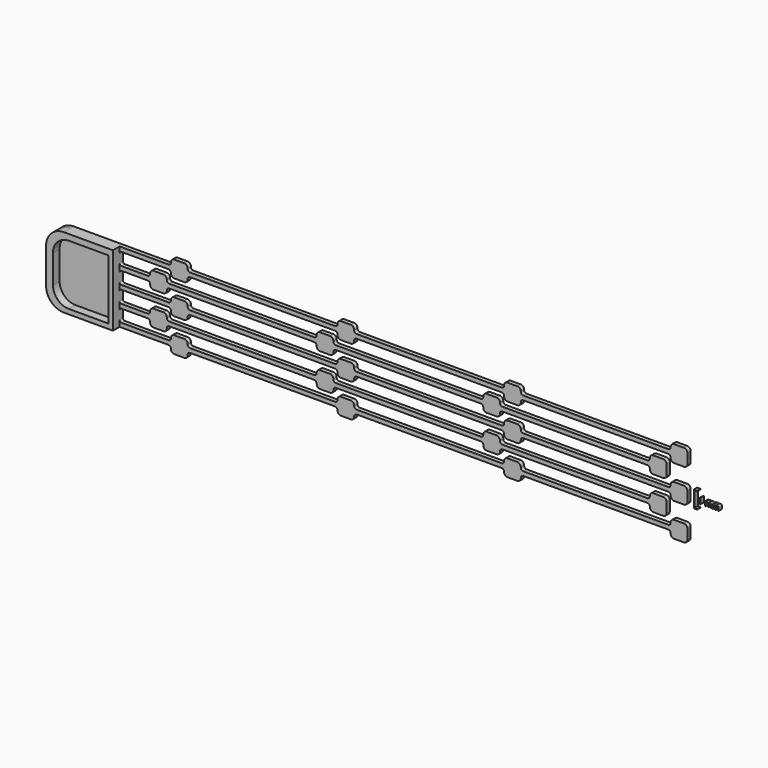
from build123d import *

# Parameters (mm, degrees)
F1_DEPTH     = 0.25
F2_W         = 0.0440478325
F2_H         = 0.0398103148
F2_W_2       = 0.1596286893
F2_H_2       = 0.9191203862
F2_H_3       = 0.0411942601
F2_TEXT_SIZE = 0.4795742118
F3_DEPTH     = 0.25
F5_DEPTH     = 0.5
F7_DEPTH     = 0.5


# Not quite as in the source:
# - ends of sketch curves that miss each other by under 0.0002 mm in the source are joined
# - Text() gives the source's letters only with a copy of the font that has no kerning and outlines rounded to 1/6400 em; it was checked with that copy


with BuildPart() as f1:
    # F0 (on Front) → F1 (new body)
    with BuildSketch(Plane.XZ):
        with BuildLine():
            ThreePointArc((50.7212476134, 27.8172210783), (50.6626689697, 27.9586424345), (50.5212476134, 28.0172210783))
            Line((50.5212476134, 28.0172210783), (49.9212476134, 28.0172210783))
            ThreePointArc((49.9212476134, 28.0172210783), (49.7798262572, 27.9586424345), (49.7212476134, 27.8172210783))
            Line((49.7212476134, 27.8172210783), (49.7212476134, 27.7922210783))
            ThreePointArc((49.7212476134, 27.7922210783), (49.6773136306, 27.6861550611), (49.5712476134, 27.6422210783))
            Line((49.5712476134, 27.6422210783), (49.1332476134, 27.6422210783))
            Line((49.1332476134, 27.6422210783), (47.8865653276, 27.6422210783))
            Line((47.8865653276, 27.6422210783), (46.7647824857, 27.6422210783))
            ThreePointArc((46.7647824857, 27.6422210783), (46.6741192638, 27.6797750144), (46.6365653276, 27.7704382363))
            Line((46.6365653276, 27.7704382363), (46.6365653276, 28.2640039202))
            ThreePointArc((46.6365653276, 28.2640039202), (46.6741192638, 28.3546671421), (46.7647824857, 28.3922210783))
            Line((46.7647824857, 28.3922210783), (47.8865653276, 28.3922210783))
            Line((47.8865653276, 28.3922210783), (48.3212476134, 28.3922210783))
            ThreePointArc((48.3212476134, 28.3922210783), (48.4273136306, 28.3482870955), (48.4712476134, 28.2422210783))
            Line((48.4712476134, 28.2422210783), (48.4712476134, 28.2172210783))
            ThreePointArc((48.4712476134, 28.2172210783), (48.5298262572, 28.075799722), (48.6712476134, 28.0172210783))
            Line((48.6712476134, 28.0172210783), (49.2712476134, 28.0172210783))
            ThreePointArc((49.2712476134, 28.0172210783), (49.4126689697, 28.075799722), (49.4712476134, 28.2172210783))
            Line((49.4712476134, 28.2172210783), (49.4712476134, 28.2422210783))
            ThreePointArc((49.4712476134, 28.2422210783), (49.5151815963, 28.3482870955), (49.6212476134, 28.3922210783))
            Line((49.6212476134, 28.3922210783), (51.1654019356, 28.3922210783))
            Line((51.1654019356, 28.3922210783), (57.8865653276, 28.3922210783))
            Line((57.8865653276, 28.3922210783), (58.3212476134, 28.3922210783))
            ThreePointArc((58.3212476134, 28.3922210783), (58.4273136306, 28.3482870955), (58.4712476134, 28.2422210783))
            Line((58.4712476134, 28.2422210783), (58.4712476134, 28.2172210783))
            ThreePointArc((58.4712476134, 28.2172210783), (58.5298262572, 28.075799722), (58.6712476134, 28.0172210783))
            Line((58.6712476134, 28.0172210783), (59.2712476134, 28.0172210783))
            ThreePointArc((59.2712476134, 28.0172210783), (59.4126689697, 28.075799722), (59.4712476134, 28.2172210783))
            Line((59.4712476134, 28.2172210783), (59.4712476134, 28.2422210783))
            ThreePointArc((59.4712476134, 28.2422210783), (59.5151815963, 28.3482870955), (59.6212476134, 28.3922210783))
            Line((59.6212476134, 28.3922210783), (61.1654019356, 28.3922210783))
            Line((61.1654019356, 28.3922210783), (67.8865653276, 28.3922210783))
            Line((67.8865653276, 28.3922210783), (68.3212476134, 28.3922210783))
            ThreePointArc((68.3212476134, 28.3922210783), (68.4273136306, 28.3482870955), (68.4712476134, 28.2422210783))
            Line((68.4712476134, 28.2422210783), (68.4712476134, 28.2172210783))
            ThreePointArc((68.4712476134, 28.2172210783), (68.5298262572, 28.075799722), (68.6712476134, 28.0172210783))
            Line((68.6712476134, 28.0172210783), (69.2712476134, 28.0172210783))
            ThreePointArc((69.2712476134, 28.0172210783), (69.4126689697, 28.075799722), (69.4712476134, 28.2172210783))
            Line((69.4712476134, 28.2172210783), (69.4712476134, 28.2422210783))
            ThreePointArc((69.4712476134, 28.2422210783), (69.5151815963, 28.3482870955), (69.6212476134, 28.3922210783))
            Line((69.6212476134, 28.3922210783), (71.1654019356, 28.3922210783))
            Line((71.1654019356, 28.3922210783), (77.8865653276, 28.3922210783))
            Line((77.8865653276, 28.3922210783), (78.3212476134, 28.3922210783))
            ThreePointArc((78.3212476134, 28.3922210783), (78.4273136306, 28.3482870955), (78.4712476134, 28.2422210783))
            Line((78.4712476134, 28.2422210783), (78.4712476134, 28.2172210783))
            ThreePointArc((78.4712476134, 28.2172210783), (78.5298262572, 28.075799722), (78.6712476134, 28.0172210783))
            Line((78.6712476134, 28.0172210783), (79.2712476134, 28.0172210783))
            ThreePointArc((79.2712476134, 28.0172210783), (79.4126689697, 28.075799722), (79.4712476134, 28.2172210783))
            Line((79.4712476134, 28.2172210783), (79.4712476134, 28.2422210783))
            Line((79.4712476134, 28.2422210783), (79.4712476134, 28.7922210783))
            Line((79.4712476134, 28.7922210783), (79.4712476134, 28.8172210783))
            ThreePointArc((79.4712476134, 28.8172210783), (79.4126689697, 28.9586424345), (79.2712476134, 29.0172210783))
            Line((79.2712476134, 29.0172210783), (78.6712476134, 29.0172210783))
            ThreePointArc((78.6712476134, 29.0172210783), (78.5298262572, 28.9586424345), (78.4712476134, 28.8172210783))
            Line((78.4712476134, 28.8172210783), (78.4712476134, 28.7922210783))
            ThreePointArc((78.4712476134, 28.7922210783), (78.4273136306, 28.6861550611), (78.3212476134, 28.6422210783))
            Line((78.3212476134, 28.6422210783), (77.8865653276, 28.6422210783))
            Line((77.8865653276, 28.6422210783), (71.1654019356, 28.6422210783))
            Line((71.1654019356, 28.6422210783), (69.6212476134, 28.6422210783))
            ThreePointArc((69.6212476134, 28.6422210783), (69.5151815963, 28.6861550611), (69.4712476134, 28.7922210783))
            Line((69.4712476134, 28.7922210783), (69.4712476134, 28.8172210783))
            ThreePointArc((69.4712476134, 28.8172210783), (69.4126689697, 28.9586424345), (69.2712476134, 29.0172210783))
            Line((69.2712476134, 29.0172210783), (68.6712476134, 29.0172210783))
            ThreePointArc((68.6712476134, 29.0172210783), (68.5298262572, 28.9586424345), (68.4712476134, 28.8172210783))
            Line((68.4712476134, 28.8172210783), (68.4712476134, 28.7922210783))
            ThreePointArc((68.4712476134, 28.7922210783), (68.4273136306, 28.6861550611), (68.3212476134, 28.6422210783))
            Line((68.3212476134, 28.6422210783), (67.8865653276, 28.6422210783))
            Line((67.8865653276, 28.6422210783), (61.1654019356, 28.6422210783))
            Line((61.1654019356, 28.6422210783), (59.6212476134, 28.6422210783))
            ThreePointArc((59.6212476134, 28.6422210783), (59.5151815963, 28.6861550611), (59.4712476134, 28.7922210783))
            Line((59.4712476134, 28.7922210783), (59.4712476134, 28.8172210783))
            ThreePointArc((59.4712476134, 28.8172210783), (59.4126689697, 28.9586424345), (59.2712476134, 29.0172210783))
            Line((59.2712476134, 29.0172210783), (58.6712476134, 29.0172210783))
            ThreePointArc((58.6712476134, 29.0172210783), (58.5298262572, 28.9586424345), (58.4712476134, 28.8172210783))
            Line((58.4712476134, 28.8172210783), (58.4712476134, 28.7922210783))
            ThreePointArc((58.4712476134, 28.7922210783), (58.4273136306, 28.6861550611), (58.3212476134, 28.6422210783))
            Line((58.3212476134, 28.6422210783), (57.8865653276, 28.6422210783))
            Line((57.8865653276, 28.6422210783), (51.1654019356, 28.6422210783))
            Line((51.1654019356, 28.6422210783), (49.6212476134, 28.6422210783))
            ThreePointArc((49.6212476134, 28.6422210783), (49.5151815963, 28.6861550611), (49.4712476134, 28.7922210783))
            Line((49.4712476134, 28.7922210783), (49.4712476134, 28.8172210783))
            ThreePointArc((49.4712476134, 28.8172210783), (49.4126689697, 28.9586424345), (49.2712476134, 29.0172210783))
            Line((49.2712476134, 29.0172210783), (48.6712476134, 29.0172210783))
            ThreePointArc((48.6712476134, 29.0172210783), (48.5298262572, 28.9586424345), (48.4712476134, 28.8172210783))
            Line((48.4712476134, 28.8172210783), (48.4712476134, 28.7922210783))
            ThreePointArc((48.4712476134, 28.7922210783), (48.4273136306, 28.6861550611), (48.3212476134, 28.6422210783))
            Line((48.3212476134, 28.6422210783), (47.8865653276, 28.6422210783))
            Line((47.8865653276, 28.6422210783), (46.7647824857, 28.6422210783))
            ThreePointArc((46.7647824857, 28.6422210783), (46.6741192638, 28.6797750144), (46.6365653276, 28.7704382363))
            Line((46.6365653276, 28.7704382363), (46.6365653276, 29.2640039202))
            ThreePointArc((46.6365653276, 29.2640039202), (46.6741192638, 29.3546671421), (46.7647824857, 29.3922210783))
            Line((46.7647824857, 29.3922210783), (47.8865653276, 29.3922210783))
            Line((47.8865653276, 29.3922210783), (49.1332476134, 29.3922210783))
            Line((49.1332476134, 29.3922210783), (49.5712476134, 29.3922210783))
            ThreePointArc((49.5712476134, 29.3922210783), (49.6773136306, 29.3482870955), (49.7212476134, 29.2422210783))
            Line((49.7212476134, 29.2422210783), (49.7212476134, 29.2172210783))
            ThreePointArc((49.7212476134, 29.2172210783), (49.7798262572, 29.075799722), (49.9212476134, 29.0172210783))
            Line((49.9212476134, 29.0172210783), (50.5212476134, 29.0172210783))
            ThreePointArc((50.5212476134, 29.0172210783), (50.6626689697, 29.075799722), (50.7212476134, 29.2172210783))
            Line((50.7212476134, 29.2172210783), (50.7212476134, 29.2422210783))
            ThreePointArc((50.7212476134, 29.2422210783), (50.7651815963, 29.3482870955), (50.8712476134, 29.3922210783))
            Line((50.8712476134, 29.3922210783), (51.1654019356, 29.3922210783))
            Line((51.1654019356, 29.3922210783), (57.8865653276, 29.3922210783))
            Line((57.8865653276, 29.3922210783), (59.1332476134, 29.3922210783))
            Line((59.1332476134, 29.3922210783), (59.5712476134, 29.3922210783))
            ThreePointArc((59.5712476134, 29.3922210783), (59.6773136306, 29.3482870955), (59.7212476134, 29.2422210783))
            Line((59.7212476134, 29.2422210783), (59.7212476134, 29.2172210783))
            ThreePointArc((59.7212476134, 29.2172210783), (59.7798262572, 29.075799722), (59.9212476134, 29.0172210783))
            Line((59.9212476134, 29.0172210783), (60.5212476134, 29.0172210783))
            ThreePointArc((60.5212476134, 29.0172210783), (60.6626689697, 29.075799722), (60.7212476134, 29.2172210783))
            Line((60.7212476134, 29.2172210783), (60.7212476134, 29.2422210783))
            ThreePointArc((60.7212476134, 29.2422210783), (60.7651815963, 29.3482870955), (60.8712476134, 29.3922210783))
            Line((60.8712476134, 29.3922210783), (61.1654019356, 29.3922210783))
            Line((61.1654019356, 29.3922210783), (67.8865653276, 29.3922210783))
            Line((67.8865653276, 29.3922210783), (69.1332476134, 29.3922210783))
            Line((69.1332476134, 29.3922210783), (69.5712476134, 29.3922210783))
            ThreePointArc((69.5712476134, 29.3922210783), (69.6773136306, 29.3482870955), (69.7212476134, 29.2422210783))
            Line((69.7212476134, 29.2422210783), (69.7212476134, 29.2172210783))
            ThreePointArc((69.7212476134, 29.2172210783), (69.7798262572, 29.075799722), (69.9212476134, 29.0172210783))
            Line((69.9212476134, 29.0172210783), (70.5212476134, 29.0172210783))
            ThreePointArc((70.5212476134, 29.0172210783), (70.6626689697, 29.075799722), (70.7212476134, 29.2172210783))
            Line((70.7212476134, 29.2172210783), (70.7212476134, 29.2422210783))
            ThreePointArc((70.7212476134, 29.2422210783), (70.7651815963, 29.3482870955), (70.8712476134, 29.3922210783))
            Line((70.8712476134, 29.3922210783), (71.1654019356, 29.3922210783))
            Line((71.1654019356, 29.3922210783), (77.8865653276, 29.3922210783))
            Line((77.8865653276, 29.3922210783), (79.1332476134, 29.3922210783))
            Line((79.1332476134, 29.3922210783), (79.5712476134, 29.3922210783))
            ThreePointArc((79.5712476134, 29.3922210783), (79.6773136306, 29.3482870955), (79.7212476134, 29.2422210783))
            Line((79.7212476134, 29.2422210783), (79.7212476134, 29.2172210783))
            ThreePointArc((79.7212476134, 29.2172210783), (79.7798262572, 29.075799722), (79.9212476134, 29.0172210783))
            Line((79.9212476134, 29.0172210783), (80.5212476134, 29.0172210783))
            ThreePointArc((80.5212476134, 29.0172210783), (80.6626689697, 29.075799722), (80.7212476134, 29.2172210783))
            Line((80.7212476134, 29.2172210783), (80.7212476134, 29.2422210783))
            Line((80.7212476134, 29.2422210783), (80.7212476134, 29.7922210783))
            Line((80.7212476134, 29.7922210783), (80.7212476134, 29.8172210783))
            ThreePointArc((80.7212476134, 29.8172210783), (80.6626689697, 29.9586424345), (80.5212476134, 30.0172210783))
            Line((80.5212476134, 30.0172210783), (79.9212476134, 30.0172210783))
            ThreePointArc((79.9212476134, 30.0172210783), (79.7798262572, 29.9586424345), (79.7212476134, 29.8172210783))
            Line((79.7212476134, 29.8172210783), (79.7212476134, 29.7922210783))
            ThreePointArc((79.7212476134, 29.7922210783), (79.6773136306, 29.6861550611), (79.5712476134, 29.6422210783))
            Line((79.5712476134, 29.6422210783), (79.1332476134, 29.6422210783))
            Line((79.1332476134, 29.6422210783), (77.8865653276, 29.6422210783))
            Line((77.8865653276, 29.6422210783), (71.1654019356, 29.6422210783))
            Line((71.1654019356, 29.6422210783), (70.8712476134, 29.6422210783))
            ThreePointArc((70.8712476134, 29.6422210783), (70.7651815963, 29.6861550611), (70.7212476134, 29.7922210783))
            Line((70.7212476134, 29.7922210783), (70.7212476134, 29.8172210783))
            ThreePointArc((70.7212476134, 29.8172210783), (70.6626689697, 29.9586424345), (70.5212476134, 30.0172210783))
            Line((70.5212476134, 30.0172210783), (69.9212476134, 30.0172210783))
            ThreePointArc((69.9212476134, 30.0172210783), (69.7798262572, 29.9586424345), (69.7212476134, 29.8172210783))
            Line((69.7212476134, 29.8172210783), (69.7212476134, 29.7922210783))
            ThreePointArc((69.7212476134, 29.7922210783), (69.6773136306, 29.6861550611), (69.5712476134, 29.6422210783))
            Line((69.5712476134, 29.6422210783), (69.1332476134, 29.6422210783))
            Line((69.1332476134, 29.6422210783), (67.8865653276, 29.6422210783))
            Line((67.8865653276, 29.6422210783), (61.1654019356, 29.6422210783))
            Line((61.1654019356, 29.6422210783), (60.8712476134, 29.6422210783))
            ThreePointArc((60.8712476134, 29.6422210783), (60.7651815963, 29.6861550611), (60.7212476134, 29.7922210783))
            Line((60.7212476134, 29.7922210783), (60.7212476134, 29.8172210783))
            ThreePointArc((60.7212476134, 29.8172210783), (60.6626689697, 29.9586424345), (60.5212476134, 30.0172210783))
            Line((60.5212476134, 30.0172210783), (59.9212476134, 30.0172210783))
            ThreePointArc((59.9212476134, 30.0172210783), (59.7798262572, 29.9586424345), (59.7212476134, 29.8172210783))
            Line((59.7212476134, 29.8172210783), (59.7212476134, 29.7922210783))
            ThreePointArc((59.7212476134, 29.7922210783), (59.6773136306, 29.6861550611), (59.5712476134, 29.6422210783))
            Line((59.5712476134, 29.6422210783), (59.1332476134, 29.6422210783))
            Line((59.1332476134, 29.6422210783), (57.8865653276, 29.6422210783))
            Line((57.8865653276, 29.6422210783), (51.1654019356, 29.6422210783))
            Line((51.1654019356, 29.6422210783), (50.8712476134, 29.6422210783))
            ThreePointArc((50.8712476134, 29.6422210783), (50.7651815963, 29.6861550611), (50.7212476134, 29.7922210783))
            Line((50.7212476134, 29.7922210783), (50.7212476134, 29.8172210783))
            ThreePointArc((50.7212476134, 29.8172210783), (50.6626689697, 29.9586424345), (50.5212476134, 30.0172210783))
            Line((50.5212476134, 30.0172210783), (49.9212476134, 30.0172210783))
            ThreePointArc((49.9212476134, 30.0172210783), (49.7798262572, 29.9586424345), (49.7212476134, 29.8172210783))
            Line((49.7212476134, 29.8172210783), (49.7212476134, 29.7922210783))
            ThreePointArc((49.7212476134, 29.7922210783), (49.6773136306, 29.6861550611), (49.5712476134, 29.6422210783))
            Line((49.5712476134, 29.6422210783), (49.1332476134, 29.6422210783))
            Line((49.1332476134, 29.6422210783), (47.8865653276, 29.6422210783))
            Line((47.8865653276, 29.6422210783), (46.7647824857, 29.6422210783))
            ThreePointArc((46.7647824857, 29.6422210783), (46.6741192638, 29.6797750144), (46.6365653276, 29.7704382363))
            Line((46.6365653276, 29.7704382363), (46.6365653276, 30.2640039202))
            ThreePointArc((46.6365653276, 30.2640039202), (46.6741192638, 30.3546671421), (46.7647824857, 30.3922210783))
            Line((46.7647824857, 30.3922210783), (47.8865653276, 30.3922210783))
            Line((47.8865653276, 30.3922210783), (48.3212476134, 30.3922210783))
            ThreePointArc((48.3212476134, 30.3922210783), (48.4273136306, 30.3482870955), (48.4712476134, 30.2422210783))
            Line((48.4712476134, 30.2422210783), (48.4712476134, 30.2172210783))
            ThreePointArc((48.4712476134, 30.2172210783), (48.5298262572, 30.075799722), (48.6712476134, 30.0172210783))
            Line((48.6712476134, 30.0172210783), (49.2712476134, 30.0172210783))
            ThreePointArc((49.2712476134, 30.0172210783), (49.4126689697, 30.075799722), (49.4712476134, 30.2172210783))
            Line((49.4712476134, 30.2172210783), (49.4712476134, 30.2422210783))
            ThreePointArc((49.4712476134, 30.2422210783), (49.5151815963, 30.3482870955), (49.6212476134, 30.3922210783))
            Line((49.6212476134, 30.3922210783), (51.1654019356, 30.3922210783))
            Line((51.1654019356, 30.3922210783), (57.8865653276, 30.3922210783))
            Line((57.8865653276, 30.3922210783), (58.3212476134, 30.3922210783))
            ThreePointArc((58.3212476134, 30.3922210783), (58.4273136306, 30.3482870955), (58.4712476134, 30.2422210783))
            Line((58.4712476134, 30.2422210783), (58.4712476134, 30.2172210783))
            ThreePointArc((58.4712476134, 30.2172210783), (58.5298262572, 30.075799722), (58.6712476134, 30.0172210783))
            Line((58.6712476134, 30.0172210783), (59.2712476134, 30.0172210783))
            ThreePointArc((59.2712476134, 30.0172210783), (59.4126689697, 30.075799722), (59.4712476134, 30.2172210783))
            Line((59.4712476134, 30.2172210783), (59.4712476134, 30.2422210783))
            ThreePointArc((59.4712476134, 30.2422210783), (59.5151815963, 30.3482870955), (59.6212476134, 30.3922210783))
            Line((59.6212476134, 30.3922210783), (61.1654019356, 30.3922210783))
            Line((61.1654019356, 30.3922210783), (67.8865653276, 30.3922210783))
            Line((67.8865653276, 30.3922210783), (68.3212476134, 30.3922210783))
            ThreePointArc((68.3212476134, 30.3922210783), (68.4273136306, 30.3482870955), (68.4712476134, 30.2422210783))
            Line((68.4712476134, 30.2422210783), (68.4712476134, 30.2172210783))
            ThreePointArc((68.4712476134, 30.2172210783), (68.5298262572, 30.075799722), (68.6712476134, 30.0172210783))
            Line((68.6712476134, 30.0172210783), (69.2712476134, 30.0172210783))
            ThreePointArc((69.2712476134, 30.0172210783), (69.4126689697, 30.075799722), (69.4712476134, 30.2172210783))
            Line((69.4712476134, 30.2172210783), (69.4712476134, 30.2422210783))
            ThreePointArc((69.4712476134, 30.2422210783), (69.5151815963, 30.3482870955), (69.6212476134, 30.3922210783))
            Line((69.6212476134, 30.3922210783), (71.1654019356, 30.3922210783))
            Line((71.1654019356, 30.3922210783), (77.8865653276, 30.3922210783))
            Line((77.8865653276, 30.3922210783), (78.3212476134, 30.3922210783))
            ThreePointArc((78.3212476134, 30.3922210783), (78.4273136306, 30.3482870955), (78.4712476134, 30.2422210783))
            Line((78.4712476134, 30.2422210783), (78.4712476134, 30.2172210783))
            ThreePointArc((78.4712476134, 30.2172210783), (78.5298262572, 30.075799722), (78.6712476134, 30.0172210783))
            Line((78.6712476134, 30.0172210783), (79.2712476134, 30.0172210783))
            ThreePointArc((79.2712476134, 30.0172210783), (79.4126689697, 30.075799722), (79.4712476134, 30.2172210783))
            Line((79.4712476134, 30.2172210783), (79.4712476134, 30.2422210783))
            Line((79.4712476134, 30.2422210783), (79.4712476134, 30.7922210783))
            Line((79.4712476134, 30.7922210783), (79.4712476134, 30.8172210783))
            ThreePointArc((79.4712476134, 30.8172210783), (79.4126689697, 30.9586424345), (79.2712476134, 31.0172210783))
            Line((79.2712476134, 31.0172210783), (78.6712476134, 31.0172210783))
            ThreePointArc((78.6712476134, 31.0172210783), (78.5298262572, 30.9586424345), (78.4712476134, 30.8172210783))
            Line((78.4712476134, 30.8172210783), (78.4712476134, 30.7922210783))
            ThreePointArc((78.4712476134, 30.7922210783), (78.4273136306, 30.6861550611), (78.3212476134, 30.6422210783))
            Line((78.3212476134, 30.6422210783), (77.8865653276, 30.6422210783))
            Line((77.8865653276, 30.6422210783), (71.1654019356, 30.6422210783))
            Line((71.1654019356, 30.6422210783), (69.6212476134, 30.6422210783))
            ThreePointArc((69.6212476134, 30.6422210783), (69.5151815963, 30.6861550611), (69.4712476134, 30.7922210783))
            Line((69.4712476134, 30.7922210783), (69.4712476134, 30.8172210783))
            ThreePointArc((69.4712476134, 30.8172210783), (69.4126689697, 30.9586424345), (69.2712476134, 31.0172210783))
            Line((69.2712476134, 31.0172210783), (68.6712476134, 31.0172210783))
            ThreePointArc((68.6712476134, 31.0172210783), (68.5298262572, 30.9586424345), (68.4712476134, 30.8172210783))
            Line((68.4712476134, 30.8172210783), (68.4712476134, 30.7922210783))
            ThreePointArc((68.4712476134, 30.7922210783), (68.4273136306, 30.6861550611), (68.3212476134, 30.6422210783))
            Line((68.3212476134, 30.6422210783), (67.8865653276, 30.6422210783))
            Line((67.8865653276, 30.6422210783), (61.1654019356, 30.6422210783))
            Line((61.1654019356, 30.6422210783), (59.6212476134, 30.6422210783))
            ThreePointArc((59.6212476134, 30.6422210783), (59.5151815963, 30.6861550611), (59.4712476134, 30.7922210783))
            Line((59.4712476134, 30.7922210783), (59.4712476134, 30.8172210783))
            ThreePointArc((59.4712476134, 30.8172210783), (59.4126689697, 30.9586424345), (59.2712476134, 31.0172210783))
            Line((59.2712476134, 31.0172210783), (58.6712476134, 31.0172210783))
            ThreePointArc((58.6712476134, 31.0172210783), (58.5298262572, 30.9586424345), (58.4712476134, 30.8172210783))
            Line((58.4712476134, 30.8172210783), (58.4712476134, 30.7922210783))
            ThreePointArc((58.4712476134, 30.7922210783), (58.4273136306, 30.6861550611), (58.3212476134, 30.6422210783))
            Line((58.3212476134, 30.6422210783), (57.8865653276, 30.6422210783))
            Line((57.8865653276, 30.6422210783), (51.1654019356, 30.6422210783))
            Line((51.1654019356, 30.6422210783), (49.6212476134, 30.6422210783))
            ThreePointArc((49.6212476134, 30.6422210783), (49.5151815963, 30.6861550611), (49.4712476134, 30.7922210783))
            Line((49.4712476134, 30.7922210783), (49.4712476134, 30.8172210783))
            ThreePointArc((49.4712476134, 30.8172210783), (49.4126689697, 30.9586424345), (49.2712476134, 31.0172210783))
            Line((49.2712476134, 31.0172210783), (48.6712476134, 31.0172210783))
            ThreePointArc((48.6712476134, 31.0172210783), (48.5298262572, 30.9586424345), (48.4712476134, 30.8172210783))
            Line((48.4712476134, 30.8172210783), (48.4712476134, 30.7922210783))
            ThreePointArc((48.4712476134, 30.7922210783), (48.4273136306, 30.6861550611), (48.3212476134, 30.6422210783))
            Line((48.3212476134, 30.6422210783), (47.8865653276, 30.6422210783))
            Line((47.8865653276, 30.6422210783), (46.7647824857, 30.6422210783))
            ThreePointArc((46.7647824857, 30.6422210783), (46.6741192638, 30.6797750144), (46.6365653276, 30.7704382363))
            Line((46.6365653276, 30.7704382363), (46.6365653276, 31.2640039202))
            ThreePointArc((46.6365653276, 31.2640039202), (46.6741192638, 31.3546671421), (46.7647824857, 31.3922210783))
            Line((46.7647824857, 31.3922210783), (47.8865653276, 31.3922210783))
            Line((47.8865653276, 31.3922210783), (49.1332476134, 31.3922210783))
            Line((49.1332476134, 31.3922210783), (49.5712476134, 31.3922210783))
            ThreePointArc((49.5712476134, 31.3922210783), (49.6773136306, 31.3482870955), (49.7212476134, 31.2422210783))
            Line((49.7212476134, 31.2422210783), (49.7212476134, 31.2172210783))
            ThreePointArc((49.7212476134, 31.2172210783), (49.7798262572, 31.075799722), (49.9212476134, 31.0172210783))
            Line((49.9212476134, 31.0172210783), (50.5212476134, 31.0172210783))
            ThreePointArc((50.5212476134, 31.0172210783), (50.6626689697, 31.075799722), (50.7212476134, 31.2172210783))
            Line((50.7212476134, 31.2172210783), (50.7212476134, 31.2422210783))
            ThreePointArc((50.7212476134, 31.2422210783), (50.7651815963, 31.3482870955), (50.8712476134, 31.3922210783))
            Line((50.8712476134, 31.3922210783), (51.1654019356, 31.3922210783))
            Line((51.1654019356, 31.3922210783), (57.8865653276, 31.3922210783))
            Line((57.8865653276, 31.3922210783), (59.1332476134, 31.3922210783))
            Line((59.1332476134, 31.3922210783), (59.5712476134, 31.3922210783))
            ThreePointArc((59.5712476134, 31.3922210783), (59.6773136306, 31.3482870955), (59.7212476134, 31.2422210783))
            Line((59.7212476134, 31.2422210783), (59.7212476134, 31.2172210783))
            ThreePointArc((59.7212476134, 31.2172210783), (59.7798262572, 31.075799722), (59.9212476134, 31.0172210783))
            Line((59.9212476134, 31.0172210783), (60.5212476134, 31.0172210783))
            ThreePointArc((60.5212476134, 31.0172210783), (60.6626689697, 31.075799722), (60.7212476134, 31.2172210783))
            Line((60.7212476134, 31.2172210783), (60.7212476134, 31.2422210783))
            ThreePointArc((60.7212476134, 31.2422210783), (60.7651815963, 31.3482870955), (60.8712476134, 31.3922210783))
            Line((60.8712476134, 31.3922210783), (61.1654019356, 31.3922210783))
            Line((61.1654019356, 31.3922210783), (67.8865653276, 31.3922210783))
            Line((67.8865653276, 31.3922210783), (69.1332476134, 31.3922210783))
            Line((69.1332476134, 31.3922210783), (69.5712476134, 31.3922210783))
            ThreePointArc((69.5712476134, 31.3922210783), (69.6773136306, 31.3482870955), (69.7212476134, 31.2422210783))
            Line((69.7212476134, 31.2422210783), (69.7212476134, 31.2172210783))
            ThreePointArc((69.7212476134, 31.2172210783), (69.7798262572, 31.075799722), (69.9212476134, 31.0172210783))
            Line((69.9212476134, 31.0172210783), (70.5212476134, 31.0172210783))
            ThreePointArc((70.5212476134, 31.0172210783), (70.6626689697, 31.075799722), (70.7212476134, 31.2172210783))
            Line((70.7212476134, 31.2172210783), (70.7212476134, 31.2422210783))
            ThreePointArc((70.7212476134, 31.2422210783), (70.7651815963, 31.3482870955), (70.8712476134, 31.3922210783))
            Line((70.8712476134, 31.3922210783), (71.1654019356, 31.3922210783))
            Line((71.1654019356, 31.3922210783), (77.8865653276, 31.3922210783))
            Line((77.8865653276, 31.3922210783), (79.1332476134, 31.3922210783))
            Line((79.1332476134, 31.3922210783), (79.5712476134, 31.3922210783))
            ThreePointArc((79.5712476134, 31.3922210783), (79.6773136306, 31.3482870955), (79.7212476134, 31.2422210783))
            Line((79.7212476134, 31.2422210783), (79.7212476134, 31.2172210783))
            ThreePointArc((79.7212476134, 31.2172210783), (79.7798262572, 31.075799722), (79.9212476134, 31.0172210783))
            Line((79.9212476134, 31.0172210783), (80.5212476134, 31.0172210783))
            ThreePointArc((80.5212476134, 31.0172210783), (80.6626689697, 31.075799722), (80.7212476134, 31.2172210783))
            Line((80.7212476134, 31.2172210783), (80.7212476134, 31.2422210783))
            Line((80.7212476134, 31.2422210783), (80.7212476134, 31.7922210783))
            Line((80.7212476134, 31.7922210783), (80.7212476134, 31.8172210783))
            ThreePointArc((80.7212476134, 31.8172210783), (80.6626689697, 31.9586424345), (80.5212476134, 32.0172210783))
            Line((80.5212476134, 32.0172210783), (79.9212476134, 32.0172210783))
            ThreePointArc((79.9212476134, 32.0172210783), (79.7798262572, 31.9586424345), (79.7212476134, 31.8172210783))
            Line((79.7212476134, 31.8172210783), (79.7212476134, 31.7922210783))
            ThreePointArc((79.7212476134, 31.7922210783), (79.6773136306, 31.6861550611), (79.5712476134, 31.6422210783))
            Line((79.5712476134, 31.6422210783), (79.1332476134, 31.6422210783))
            Line((79.1332476134, 31.6422210783), (77.8865653276, 31.6422210783))
            Line((77.8865653276, 31.6422210783), (71.1654019356, 31.6422210783))
            Line((71.1654019356, 31.6422210783), (70.8712476134, 31.6422210783))
            ThreePointArc((70.8712476134, 31.6422210783), (70.7651815963, 31.6861550611), (70.7212476134, 31.7922210783))
            Line((70.7212476134, 31.7922210783), (70.7212476134, 31.8172210783))
            ThreePointArc((70.7212476134, 31.8172210783), (70.6626689697, 31.9586424345), (70.5212476134, 32.0172210783))
            Line((70.5212476134, 32.0172210783), (69.9212476134, 32.0172210783))
            ThreePointArc((69.9212476134, 32.0172210783), (69.7798262572, 31.9586424345), (69.7212476134, 31.8172210783))
            Line((69.7212476134, 31.8172210783), (69.7212476134, 31.7922210783))
            ThreePointArc((69.7212476134, 31.7922210783), (69.6773136306, 31.6861550611), (69.5712476134, 31.6422210783))
            Line((69.5712476134, 31.6422210783), (69.1332476134, 31.6422210783))
            Line((69.1332476134, 31.6422210783), (67.8865653276, 31.6422210783))
            Line((67.8865653276, 31.6422210783), (61.1654019356, 31.6422210783))
            Line((61.1654019356, 31.6422210783), (60.8712476134, 31.6422210783))
            ThreePointArc((60.8712476134, 31.6422210783), (60.7651815963, 31.6861550611), (60.7212476134, 31.7922210783))
            Line((60.7212476134, 31.7922210783), (60.7212476134, 31.8172210783))
            ThreePointArc((60.7212476134, 31.8172210783), (60.6626689697, 31.9586424345), (60.5212476134, 32.0172210783))
            Line((60.5212476134, 32.0172210783), (59.9212476134, 32.0172210783))
            ThreePointArc((59.9212476134, 32.0172210783), (59.7798262572, 31.9586424345), (59.7212476134, 31.8172210783))
            Line((59.7212476134, 31.8172210783), (59.7212476134, 31.7922210783))
            ThreePointArc((59.7212476134, 31.7922210783), (59.6773136306, 31.6861550611), (59.5712476134, 31.6422210783))
            Line((59.5712476134, 31.6422210783), (59.1332476134, 31.6422210783))
            Line((59.1332476134, 31.6422210783), (57.8865653276, 31.6422210783))
            Line((57.8865653276, 31.6422210783), (51.1654019356, 31.6422210783))
            Line((51.1654019356, 31.6422210783), (50.8712476134, 31.6422210783))
            ThreePointArc((50.8712476134, 31.6422210783), (50.7651815963, 31.6861550611), (50.7212476134, 31.7922210783))
            Line((50.7212476134, 31.7922210783), (50.7212476134, 31.8172210783))
            ThreePointArc((50.7212476134, 31.8172210783), (50.6626689697, 31.9586424345), (50.5212476134, 32.0172210783))
            Line((50.5212476134, 32.0172210783), (49.9212476134, 32.0172210783))
            ThreePointArc((49.9212476134, 32.0172210783), (49.7798262572, 31.9586424345), (49.7212476134, 31.8172210783))
            Line((49.7212476134, 31.8172210783), (49.7212476134, 31.7922210783))
            ThreePointArc((49.7212476134, 31.7922210783), (49.6773136306, 31.6861550611), (49.5712476134, 31.6422210783))
            Line((49.5712476134, 31.6422210783), (49.1332476134, 31.6422210783))
            Line((49.1332476134, 31.6422210783), (47.8865653276, 31.6422210783))
            Line((47.8865653276, 31.6422210783), (43.6902402822, 31.6422210783))
            ThreePointArc((43.6902402822, 31.6422210783), (42.9369955648, 31.3302169006), (42.6249913871, 30.5769721832))
            Line((42.6249913871, 30.5769721832), (42.6249913871, 28.4574699733))
            ThreePointArc((42.6249913871, 28.4574699733), (42.9369955648, 27.704225256), (43.6902402822, 27.3922210783))
            Line((43.6902402822, 27.3922210783), (47.8865653276, 27.3922210783))
            Line((47.8865653276, 27.3922210783), (49.1332476134, 27.3922210783))
            Line((49.1332476134, 27.3922210783), (49.5712476134, 27.3922210783))
            ThreePointArc((49.5712476134, 27.3922210783), (49.6773136306, 27.3482870955), (49.7212476134, 27.2422210783))
            Line((49.7212476134, 27.2422210783), (49.7212476134, 27.2172210783))
            ThreePointArc((49.7212476134, 27.2172210783), (49.7798262572, 27.075799722), (49.9212476134, 27.0172210783))
            Line((49.9212476134, 27.0172210783), (50.5212476134, 27.0172210783))
            ThreePointArc((50.5212476134, 27.0172210783), (50.6626689697, 27.075799722), (50.7212476134, 27.2172210783))
            Line((50.7212476134, 27.2172210783), (50.7212476134, 27.2422210783))
            ThreePointArc((50.7212476134, 27.2422210783), (50.7651815963, 27.3482870955), (50.8712476134, 27.3922210783))
            Line((50.8712476134, 27.3922210783), (51.1654019356, 27.3922210783))
            Line((51.1654019356, 27.3922210783), (57.8865653276, 27.3922210783))
            Line((57.8865653276, 27.3922210783), (59.1332476134, 27.3922210783))
            Line((59.1332476134, 27.3922210783), (59.5712476134, 27.3922210783))
            ThreePointArc((59.5712476134, 27.3922210783), (59.6773136306, 27.3482870955), (59.7212476134, 27.2422210783))
            Line((59.7212476134, 27.2422210783), (59.7212476134, 27.2172210783))
            ThreePointArc((59.7212476134, 27.2172210783), (59.7798262572, 27.075799722), (59.9212476134, 27.0172210783))
            Line((59.9212476134, 27.0172210783), (60.5212476134, 27.0172210783))
            ThreePointArc((60.5212476134, 27.0172210783), (60.6626689697, 27.075799722), (60.7212476134, 27.2172210783))
            Line((60.7212476134, 27.2172210783), (60.7212476134, 27.2422210783))
            ThreePointArc((60.7212476134, 27.2422210783), (60.7651815963, 27.3482870955), (60.8712476134, 27.3922210783))
            Line((60.8712476134, 27.3922210783), (61.1654019356, 27.3922210783))
            Line((61.1654019356, 27.3922210783), (67.8865653276, 27.3922210783))
            Line((67.8865653276, 27.3922210783), (69.1332476134, 27.3922210783))
            Line((69.1332476134, 27.3922210783), (69.5712476134, 27.3922210783))
            ThreePointArc((69.5712476134, 27.3922210783), (69.6773136306, 27.3482870955), (69.7212476134, 27.2422210783))
            Line((69.7212476134, 27.2422210783), (69.7212476134, 27.2172210783))
            ThreePointArc((69.7212476134, 27.2172210783), (69.7798262572, 27.075799722), (69.9212476134, 27.0172210783))
            Line((69.9212476134, 27.0172210783), (70.5212476134, 27.0172210783))
            ThreePointArc((70.5212476134, 27.0172210783), (70.6626689697, 27.075799722), (70.7212476134, 27.2172210783))
            Line((70.7212476134, 27.2172210783), (70.7212476134, 27.2422210783))
            ThreePointArc((70.7212476134, 27.2422210783), (70.7651815963, 27.3482870955), (70.8712476134, 27.3922210783))
            Line((70.8712476134, 27.3922210783), (71.1654019356, 27.3922210783))
            Line((71.1654019356, 27.3922210783), (77.8865653276, 27.3922210783))
            Line((77.8865653276, 27.3922210783), (79.1332476134, 27.3922210783))
            Line((79.1332476134, 27.3922210783), (79.5712476134, 27.3922210783))
            ThreePointArc((79.5712476134, 27.3922210783), (79.6773136306, 27.3482870955), (79.7212476134, 27.2422210783))
            Line((79.7212476134, 27.2422210783), (79.7212476134, 27.2172210783))
            ThreePointArc((79.7212476134, 27.2172210783), (79.7798262572, 27.075799722), (79.9212476134, 27.0172210783))
            Line((79.9212476134, 27.0172210783), (80.5212476134, 27.0172210783))
            ThreePointArc((80.5212476134, 27.0172210783), (80.6626689697, 27.075799722), (80.7212476134, 27.2172210783))
            Line((80.7212476134, 27.2172210783), (80.7212476134, 27.2422210783))
            Line((80.7212476134, 27.2422210783), (80.7212476134, 27.7922210783))
            Line((80.7212476134, 27.7922210783), (80.7212476134, 27.8172210783))
            ThreePointArc((80.7212476134, 27.8172210783), (80.6626689697, 27.9586424345), (80.5212476134, 28.0172210783))
            Line((80.5212476134, 28.0172210783), (79.9212476134, 28.0172210783))
            ThreePointArc((79.9212476134, 28.0172210783), (79.7798262572, 27.9586424345), (79.7212476134, 27.8172210783))
            Line((79.7212476134, 27.8172210783), (79.7212476134, 27.7922210783))
            ThreePointArc((79.7212476134, 27.7922210783), (79.6773136306, 27.6861550611), (79.5712476134, 27.6422210783))
            Line((79.5712476134, 27.6422210783), (79.1332476134, 27.6422210783))
            Line((79.1332476134, 27.6422210783), (77.8865653276, 27.6422210783))
            Line((77.8865653276, 27.6422210783), (71.1654019356, 27.6422210783))
            Line((71.1654019356, 27.6422210783), (70.8712476134, 27.6422210783))
            ThreePointArc((70.8712476134, 27.6422210783), (70.7651815963, 27.6861550611), (70.7212476134, 27.7922210783))
            Line((70.7212476134, 27.7922210783), (70.7212476134, 27.8172210783))
            ThreePointArc((70.7212476134, 27.8172210783), (70.6626689697, 27.9586424345), (70.5212476134, 28.0172210783))
            Line((70.5212476134, 28.0172210783), (69.9212476134, 28.0172210783))
            ThreePointArc((69.9212476134, 28.0172210783), (69.7798262572, 27.9586424345), (69.7212476134, 27.8172210783))
            Line((69.7212476134, 27.8172210783), (69.7212476134, 27.7922210783))
            ThreePointArc((69.7212476134, 27.7922210783), (69.6773136306, 27.6861550611), (69.5712476134, 27.6422210783))
            Line((69.5712476134, 27.6422210783), (69.1332476134, 27.6422210783))
            Line((69.1332476134, 27.6422210783), (67.8865653276, 27.6422210783))
            Line((67.8865653276, 27.6422210783), (61.1654019356, 27.6422210783))
            Line((61.1654019356, 27.6422210783), (60.8712476134, 27.6422210783))
            ThreePointArc((60.8712476134, 27.6422210783), (60.7651815963, 27.6861550611), (60.7212476134, 27.7922210783))
            Line((60.7212476134, 27.7922210783), (60.7212476134, 27.8172210783))
            ThreePointArc((60.7212476134, 27.8172210783), (60.6626689697, 27.9586424345), (60.5212476134, 28.0172210783))
            Line((60.5212476134, 28.0172210783), (59.9212476134, 28.0172210783))
            ThreePointArc((59.9212476134, 28.0172210783), (59.7798262572, 27.9586424345), (59.7212476134, 27.8172210783))
            Line((59.7212476134, 27.8172210783), (59.7212476134, 27.7922210783))
            ThreePointArc((59.7212476134, 27.7922210783), (59.6773136306, 27.6861550611), (59.5712476134, 27.6422210783))
            Line((59.5712476134, 27.6422210783), (59.1332476134, 27.6422210783))
            Line((59.1332476134, 27.6422210783), (57.8865653276, 27.6422210783))
            Line((57.8865653276, 27.6422210783), (51.1654019356, 27.6422210783))
            Line((51.1654019356, 27.6422210783), (50.8712476134, 27.6422210783))
            ThreePointArc((50.8712476134, 27.6422210783), (50.7651815963, 27.6861550611), (50.7212476134, 27.7922210783))
            Line((50.7212476134, 27.7922210783), (50.7212476134, 27.8172210783))
        make_face()
    extrude(amount=F1_DEPTH)

    # F4 (on face) → F5 (join)
    with BuildSketch(Plane.XZ.offset(0.25)):
        with BuildLine():
            Line((46.6365653276, 31.2640039202), (46.6365653276, 31.6422210783))
            Line((46.6365653276, 31.6422210783), (43.6902402822, 31.6422210783))
            Line((43.6902402822, 31.6422210783), (43.6797258529, 31.6422210783))
            ThreePointArc((43.6797258529, 31.6422210783), (42.933287461, 31.3264904518), (42.6249913871, 30.5769721832))
            Line((42.6249913871, 30.5769721832), (42.6249913871, 28.4574699733))
            ThreePointArc((42.6249913871, 28.4574699733), (42.933287461, 27.7079517048), (43.6797263651, 27.3922729653))
            Line((43.6797263651, 27.3922729653), (43.6902402822, 27.3922210783))
            Line((43.6902402822, 27.3922210783), (46.6365653276, 27.3922210783))
            Line((46.6365653276, 27.3922210783), (46.6365653276, 27.7704382363))
            Line((46.6365653276, 27.7704382363), (46.6365653276, 28.2640039202))
            Line((46.6365653276, 28.2640039202), (46.6365653276, 28.7704382363))
            Line((46.6365653276, 28.7704382363), (46.6365653276, 29.2640039202))
            Line((46.6365653276, 29.2640039202), (46.6365653276, 29.7704382363))
            Line((46.6365653276, 29.7704382363), (46.6365653276, 30.2640039202))
            Line((46.6365653276, 30.2640039202), (46.6365653276, 30.7704382363))
            Line((46.6365653276, 30.7704382363), (46.6365653276, 31.2640039202))
        make_face()
    extrude(amount=F5_DEPTH)

    # F6 (on face) → F7 (cut)
    with BuildSketch(Plane.XZ.offset(0.75)):
        with BuildLine():
            Line((46.3622398674, 27.6831910014), (46.3622398674, 31.2864722807))
            Line((46.3622398674, 31.2864722807), (43.9912102393, 31.2864722807))
            ThreePointArc((43.9912102393, 31.2864722807), (43.3149467205, 31.0063547595), (43.0348291993, 30.3300912407))
            Line((43.0348291993, 30.3300912407), (43.0348291993, 28.6395720414))
            ThreePointArc((43.0348291993, 28.6395720414), (43.3149467205, 27.9633085226), (43.9912102393, 27.6831910014))
            Line((43.9912102393, 27.6831910014), (46.3622398674, 27.6831910014))
        make_face()
    extrude(amount=-F7_DEPTH, mode=Mode.SUBTRACT)


with BuildPart() as f3:
    # F2 (on Front) → F3 (new body)
    with BuildSketch(Plane.XZ):
        with Locations((81.1283886433, 29.0266564116)):
            Rectangle(F2_W, F2_H)
        with Locations((81.2302269042, 29.0266564116)):
            Rectangle(F2_W_2, F2_H)
        with Locations((81.1283886433, 29.5061217621)):
            Rectangle(F2_W, F2_H_2)
        with Locations((81.1283886433, 29.9862790853)):
            Rectangle(F2_W, F2_H_3)
        with Locations((81.2302269042, 29.9862790853)):
            Rectangle(F2_W_2, F2_H_3)
        with Locations((81.3453942537, 29.3522607535)):
            Text('1 mm', F2_TEXT_SIZE, font='Open Sans', text_align=(TextAlign.LEFT, TextAlign.BOTTOM))
    extrude(amount=F3_DEPTH)


solid = Compound([f1.part, f3.part])
